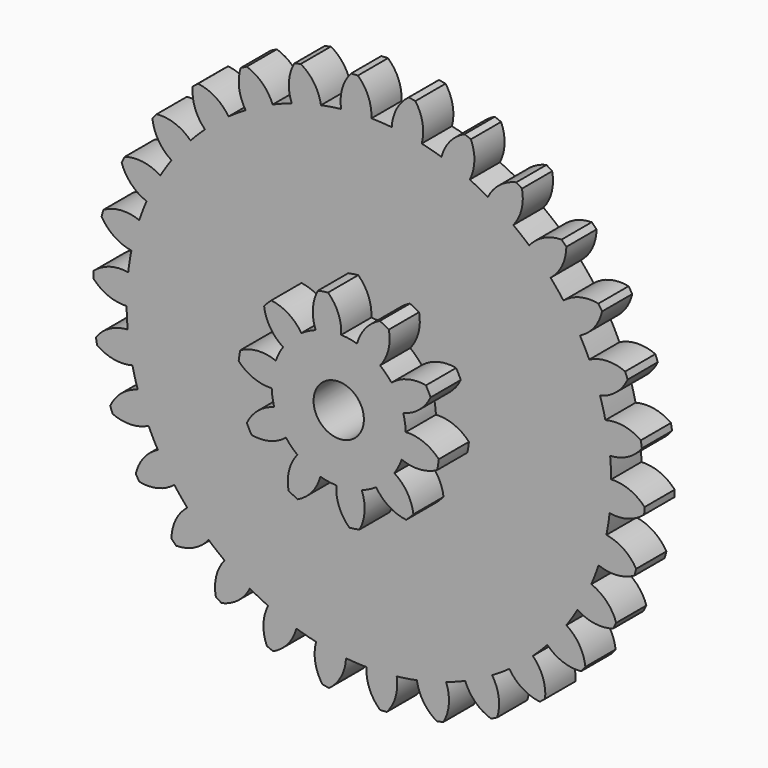
from build123d import *

# Parameters (mm, degrees)
F0_R            = 3.175
F1_DEPTH        = 4.7625
F1_COPIES_COUNT = 30
F2_R            = 3.175
F3_DEPTH        = 4.7625
F3_COPIES_COUNT = 10


# Not quite as in the source:
# - a feature of the source that left no trace in its solid (it failed there, or was rolled back) is left out
# - a pattern or mirror of a feature is missing from the dataset's text; its kind, count and spacing are read off the source's solid


with BuildPart() as f1:
    # F0 (on Front) → F1 (new body)
    with BuildSketch(Plane.XZ):
        with BuildLine():
            ThreePointArc((-3.5055458404, 30.3860678703), (-20.3516055667, -22.8344941506), (30.587611418, 0))
            ThreePointArc((30.587611418, 0), (21.7380795316, 21.5187794853), (0.3101331142, 30.5860391308))
            ThreePointArc((0.3101331142, 30.5860391308), (-1.6008318927, 30.5456921596), (-3.5055458404, 30.3860678703))
        make_face()
        Circle(F0_R, mode=Mode.SUBTRACT)
        with BuildLine():
            ThreePointArc((-3.5055458404, 30.3860678703), (-1.6008318927, 30.5456921596), (0.3101331142, 30.5860391308))
            ThreePointArc((0.3101331142, 30.5860391308), (-0.068160863, 32.8815802422), (-1.3944502868, 34.7930120855))
            ThreePointArc((-1.3944502868, 34.7930120855), (-1.822387432, 34.7732236876), (-2.2500487435, 34.7481720704))
            ThreePointArc((-2.2500487435, 34.7481720704), (-3.3692735818, 32.7085762554), (-3.5055458404, 30.3860678703))
        make_face()
    extrude(amount=F1_DEPTH)

    # F1_copies: F1 ×30 about axis
    f1_copies_axis = Axis((0, 0, 0), (0, 1, 0))


with BuildPart() as f1_1:
    add(f1.part)
    for i in range(1, F1_COPIES_COUNT):
        add(f1.part.rotate(f1_copies_axis, i * 360 / F1_COPIES_COUNT))

    # F2 (on face) → F3 (join)
    with BuildSketch(Plane.XZ.offset(4.7625)):
        with BuildLine():
            ThreePointArc((-2.909315706, 7.9511210887), (-4.8503730853, -6.9396199736), (8.4666666667, 0))
            ThreePointArc((8.4666666667, 0), (6.0954162172, 5.8762526821), (0.3098921194, 8.4609935184))
            ThreePointArc((0.3098921194, 8.4609935184), (-1.3244784707, 8.3624279504), (-2.909315706, 7.9511210887))
        make_face()
        Circle(F2_R, mode=Mode.SUBTRACT)
        with BuildLine():
            ThreePointArc((-2.909315706, 7.9511210887), (-1.3244784707, 8.3624279504), (0.3098921194, 8.4609935184))
            ThreePointArc((0.3098921194, 8.4609935184), (-0.0554250299, 10.7289090003), (-1.3473672642, 12.6283253623))
            ThreePointArc((-1.3473672642, 12.6283253623), (-1.986717706, 12.5436419256), (-2.620944731, 12.426610508))
            ThreePointArc((-2.620944731, 12.426610508), (-3.2627028763, 10.2209260937), (-2.909315706, 7.9511210887))
        make_face()
    f3 = extrude(amount=F3_DEPTH)

    # F3_copies: F3 ×10 about axis
    f3_copies_axis = Axis((0, 0, 0), (0, 1, 0))
    for i in range(1, F3_COPIES_COUNT):
        add(f3.rotate(f3_copies_axis, i * 360 / F3_COPIES_COUNT))


solid = f1_1.part
